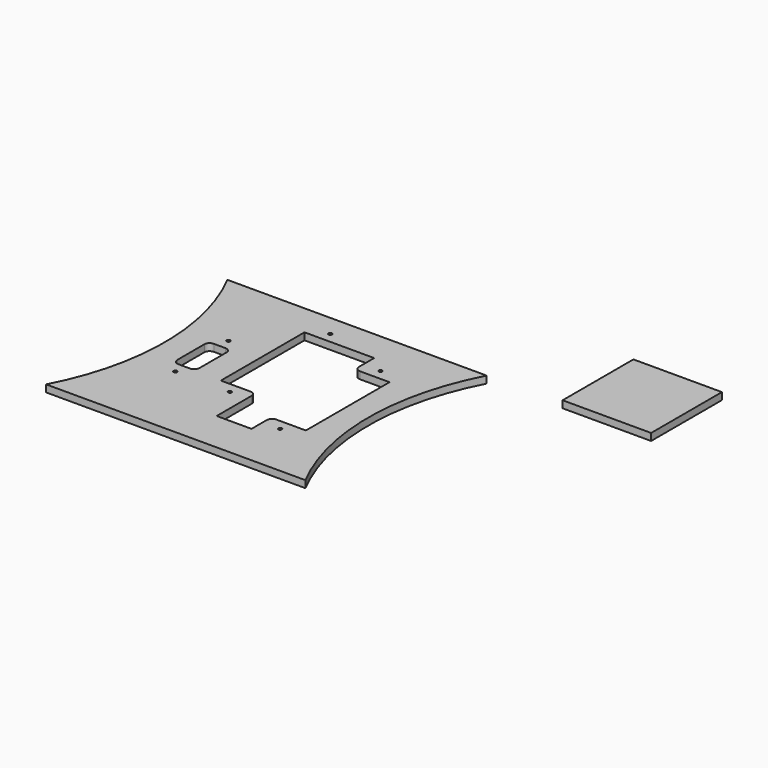
from build123d import *

# Parameters (mm, degrees)
F0_R     = 0.5
F1_DEPTH = 2.032
F0_W     = 25.4
F0_H     = 25.4


# Not quite as in the source:
# - ends of sketch curves that miss each other by under 0.0002 mm in the source are joined


with BuildPart() as f1:
    # F0 (on Top) → F1 (new body)
    with BuildSketch(Plane.XY):
        with BuildLine():
            ThreePointArc((-54.43, 32.4999997839), (-46.43, -2.161e-07), (-54.43, -32.5000002161))
            Line((-54.43, -32.5000002161), (20, -32.5000002161))
            ThreePointArc((20, -32.5000002161), (12, -2.161e-07), (20, 32.4999997839))
            Line((20, 32.4999997839), (-54.43, 32.4999997839))
        make_face()
        with Locations((-20, -9.6000002161)):
            Circle(F0_R, mode=Mode.SUBTRACT)
        with Locations((0, -16.6)):
            Circle(F0_R, mode=Mode.SUBTRACT)
        with Locations((-35.715, -9.525)):
            Circle(F0_R, mode=Mode.SUBTRACT)
        with BuildLine():
            Line((-32.54, 4.8499995679), (-32.54, -4.85))
            ThreePointArc((-32.54, -4.85), (-32.9793398282, -5.9106601718), (-34.04, -6.35))
            Line((-34.04, -6.35), (-37.39, -6.35))
            ThreePointArc((-37.39, -6.35), (-38.4506601718, -5.9106606039), (-38.89, -4.8500004321))
            Line((-38.89, -4.8500004321), (-38.89, 4.85))
            ThreePointArc((-38.89, 4.85), (-38.4506601718, 5.9106601718), (-37.39, 6.35))
            Line((-37.39, 6.35), (-34.04, 6.35))
            ThreePointArc((-34.04, 6.35), (-32.9793398282, 5.9106597396), (-32.54, 4.8499995679))
        make_face(mode=Mode.SUBTRACT)
        with Locations((-35.715, 9.5249997839)):
            Circle(F0_R, mode=Mode.SUBTRACT)
        with BuildLine():
            Line((-5, -20.6000001803), (-15, -20.6000001803))
            Line((-15, -20.6000001803), (-15, -8.1000002161))
            ThreePointArc((-15, -8.1000002161), (-15.4393398282, -7.0393400443), (-16.5, -6.6000002161))
            Line((-16.5, -6.6000002161), (-25, -6.6000002161))
            Line((-25, -6.6000002161), (-25, 23.3999996036))
            Line((-25, 23.3999996036), (-5, 23.3999996036))
            Line((-5, 23.3999996036), (-5, 17.9))
            ThreePointArc((-5, 17.9), (-4.5606601718, 16.8393398282), (-3.5, 16.4))
            Line((-3.5, 16.4), (5, 16.4))
            Line((5, 16.4), (5, -13.5999998197))
            Line((5, -13.5999998197), (-3.5, -13.6))
            ThreePointArc((-3.5, -13.6), (-4.5606601718, -14.0393398282), (-5, -15.1))
            Line((-5, -15.1), (-5, -20.6000001803))
        make_face(mode=Mode.SUBTRACT)
        with Locations((0, 19.4)):
            Circle(F0_R, mode=Mode.SUBTRACT)
        with Locations((-20, 26.3999997839)):
            Circle(F0_R, mode=Mode.SUBTRACT)
    extrude(amount=F1_DEPTH)


with BuildPart() as f1b:
    # F0 (on Top) → F1, piece 2 (new body)
    with BuildSketch(Plane.XY):
        with Locations((53.4646574736, 46.4799787521)):
            Rectangle(F0_W, F0_H)
    extrude(amount=F1_DEPTH)


solid = Compound([f1.part, f1b.part])
